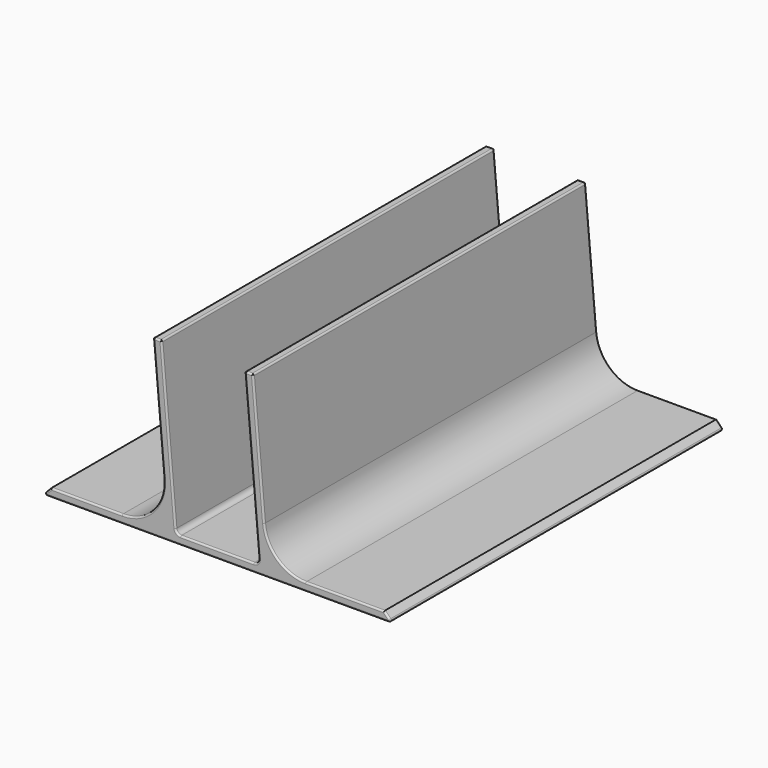
from build123d import *

# Parameters (mm, degrees)
F1_DEPTH    = 50
F2_R        = 5
F3_R        = 0.6
F4_R        = 0.2
F5_T1_DEPTH = 50.516331174
F5_T3_DEPTH = 50.6913085011


# Not quite as in the source:
# - a fillet or chamfer that OpenCascade refuses, or shapes differently, is made with other operations: its cross-section is extruded or revolved along the edge and cut away or added


with BuildPart() as f1:
    # F0 (on Front) → F1 (new body)
    with BuildSketch(Plane.XZ):
        Polygon((5, 0), (-5, 0), (-6.743114855, 19.9238939618), (-7.743114855, 19.9238939618), (-6, 0), (-20, 0), (-21, -1), (21, -1), (20, 0), (6, 0), (4.256885145, 19.9238939618), (3.256885145, 19.9238939618), align=None)
    extrude(amount=F1_DEPTH)

    # F2
    f2_edges = [f1.edges().sort_by_distance(p)[0] for p in [
        (-6, -25, 0),
        (6, -25, 0),
    ]]
    fillet(f2_edges, radius=F2_R)

    # F3
    f3_edges = [f1.edges().sort_by_distance(p)[0] for p in [
        (-5, -25, 0),
        (5, -25, 0),
    ]]
    fillet(f3_edges, radius=F3_R)

    # F4
    f4_edges = [f1.edges().sort_by_distance(p)[0] for p in [
        (-21, -25, -1),
        (21, -25, -1),
        (0, 0, -1),
        (0, -50, -1),
        (-5.895516, -50, 10.2358),
        (-4.855555, -50, 0.157634),
        (-7.243115, -50, 19.923894),
        (-0.052493, -50, 0),
        (-7.109342, -50, 12.679836),
        (4.787581, -50, 0.194646),
        (-7.770156, -50, 1.622049),
        (4.099908, -50, 10.288094),
        (-15.728271, -50, 0),
        (3.756885, -50, 19.923894),
        (-20.5, -50, -0.5),
        (4.928784, -50, 12.244058),
        (7.203705, -50, 1.313613),
        (20.5, -50, -0.5),
        (15.290828, -50, 0),
        (-5.895516, 0, 10.2358),
        (-4.855555, 0, 0.157634),
        (-7.243115, 0, 19.923894),
        (-0.052493, 0, 0),
        (-7.109342, 0, 12.679836),
        (4.787581, 0, 0.194646),
        (-7.770156, 0, 1.622049),
        (4.099908, 0, 10.288094),
        (-15.728271, 0, 0),
        (3.756885, 0, 19.923894),
        (-20.5, 0, -0.5),
        (4.928784, 0, 12.244058),
        (7.203705, 0, 1.313613),
        (20.5, 0, -0.5),
        (15.290828, 0, 0),
    ]]
    fillet(f4_edges, radius=F4_R)

    # F5: fillet of radius 0.2 on 8 edges, made by hand

    # F5_s2 → F5_t1 (cut)
    with BuildSketch(Plane.XZ.offset(-0.258165587)):
        with BuildLine():
            ThreePointArc((-6.9263810898, 19.9238939618), (-6.7912630482, 19.8713494292), (-6.7271421501, 19.7413251104))
            Line((-6.7271421501, 19.7413251104), (-6.743114855, 19.9238939618))
            Line((-6.743114855, 19.9238939618), (-6.9263810898, 19.9238939618))
        make_face()
        with BuildLine():
            ThreePointArc((4.2728578499, 19.7413251104), (4.2087369518, 19.8713494292), (4.0736189102, 19.9238939618))
            Line((4.0736189102, 19.9238939618), (4.256885145, 19.9238939618))
            Line((4.256885145, 19.9238939618), (4.2728578499, 19.7413251104))
        make_face()
    extrude(amount=F5_T1_DEPTH, mode=Mode.SUBTRACT)

    # F5_s4 → F5_t3 (cut)
    with BuildSketch(Plane.XZ.offset(-0.3456542505)):
        with BuildLine():
            ThreePointArc((-7.7240920944, 19.7064628133), (-7.6723086221, 19.8590120034), (-7.5248531547, 19.9238939618))
            Line((-7.5248531547, 19.9238939618), (-7.743114855, 19.9238939618))
            Line((-7.743114855, 19.9238939618), (-7.7240920944, 19.7064628133))
        make_face()
        with BuildLine():
            ThreePointArc((3.4751468453, 19.9238939618), (3.3276913779, 19.8590120034), (3.2759079056, 19.7064628133))
            Line((3.2759079056, 19.7064628133), (3.256885145, 19.9238939618))
            Line((3.256885145, 19.9238939618), (3.4751468453, 19.9238939618))
        make_face()
    extrude(amount=F5_T3_DEPTH, mode=Mode.SUBTRACT)


solid = f1.part
